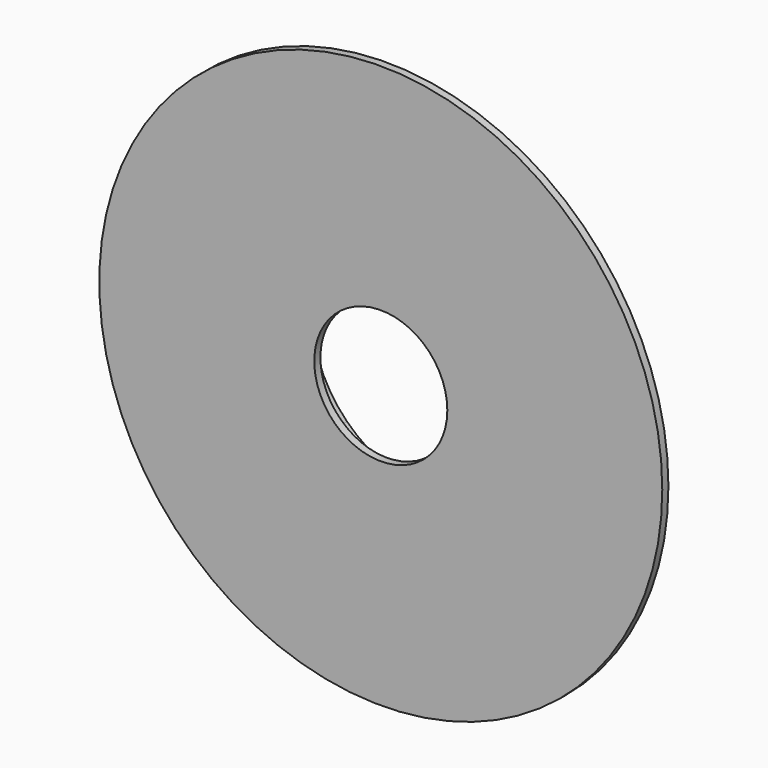
from build123d import *

# Parameters (mm, degrees)
F1_DEPTH = 22
F2_R     = 110
F2_R_2   = 50
F2_R_3   = 47
F3_DEPTH = 3
F4_R     = 26
F5_DEPTH = 3
F6_DEPTH = 25


# Not quite as in the source:
# - a feature names something its author has since deleted; it is built from what else it names


with BuildPart() as f1:
    # F0 (on Front) → F1 (new body)
    with BuildSketch(Plane.XZ):
        with BuildLine():
            Line((48.5, 0), (50, 0))
            ThreePointArc((50, 0), (46.1939766256, 19.1341716183), (35.3553390593, 35.3553390593))
            Line((35.3553390593, 35.3553390593), (34.2946788875, 34.2946788875))
            ThreePointArc((34.2946788875, 34.2946788875), (44.8081573268, 18.5601464697), (48.5, 0))
        make_face()
        with BuildLine():
            ThreePointArc((35.3553390593, -35.3553390593), (46.1939766256, -19.1341716183), (50, 0))
            Line((50, 0), (48.5, 0))
            ThreePointArc((48.5, 0), (44.8081573268, -18.5601464697), (34.2946788875, -34.2946788875))
            Line((34.2946788875, -34.2946788875), (35.3553390593, -35.3553390593))
        make_face()
        with BuildLine():
            Line((34.2946788875, 34.2946788875), (35.3553390593, 35.3553390593))
            ThreePointArc((35.3553390593, 35.3553390593), (19.1341716183, 46.1939766256), (0, 50))
            Line((0, 50), (0, 48.5))
            ThreePointArc((0, 48.5), (18.5601464697, 44.8081573268), (34.2946788875, 34.2946788875))
        make_face()
        with BuildLine():
            ThreePointArc((0, -50), (19.1341716183, -46.1939766256), (35.3553390593, -35.3553390593))
            Line((35.3553390593, -35.3553390593), (34.2946788875, -34.2946788875))
            ThreePointArc((34.2946788875, -34.2946788875), (18.5601464697, -44.8081573268), (0, -48.5))
            Line((0, -48.5), (0, -50))
        make_face()
        with BuildLine():
            Line((47, 0), (48.5, 0))
            ThreePointArc((48.5, 0), (44.8081573268, 18.5601464697), (34.2946788875, 34.2946788875))
            Line((34.2946788875, 34.2946788875), (33.2340187158, 33.2340187158))
            ThreePointArc((33.2340187158, 33.2340187158), (43.422338028, 17.9861213212), (47, 0))
        make_face()
        with BuildLine():
            ThreePointArc((34.2946788875, -34.2946788875), (44.8081573268, -18.5601464697), (48.5, 0))
            Line((48.5, 0), (47, 0))
            ThreePointArc((47, 0), (43.422338028, -17.9861213212), (33.2340187158, -33.2340187158))
            Line((33.2340187158, -33.2340187158), (34.2946788875, -34.2946788875))
        make_face()
        with BuildLine():
            Line((0, 48.5), (0, 50))
            ThreePointArc((0, 50), (-19.1341716183, 46.1939766256), (-35.3553390593, 35.3553390593))
            Line((-35.3553390593, 35.3553390593), (-34.2946788875, 34.2946788875))
            ThreePointArc((-34.2946788875, 34.2946788875), (-18.5601464697, 44.8081573268), (0, 48.5))
        make_face()
        with BuildLine():
            Line((33.2340187158, 33.2340187158), (34.2946788875, 34.2946788875))
            ThreePointArc((34.2946788875, 34.2946788875), (18.5601464697, 44.8081573268), (0, 48.5))
            Line((0, 48.5), (0, 47))
            ThreePointArc((0, 47), (17.9861213212, 43.422338028), (33.2340187158, 33.2340187158))
        make_face()
        with BuildLine():
            ThreePointArc((-35.3553390593, -35.3553390593), (-19.1341716183, -46.1939766256), (0, -50))
            Line((0, -50), (0, -48.5))
            ThreePointArc((0, -48.5), (-18.5601464697, -44.8081573268), (-34.2946788875, -34.2946788875))
            Line((-34.2946788875, -34.2946788875), (-35.3553390593, -35.3553390593))
        make_face()
        with BuildLine():
            ThreePointArc((0, -48.5), (18.5601464697, -44.8081573268), (34.2946788875, -34.2946788875))
            Line((34.2946788875, -34.2946788875), (33.2340187158, -33.2340187158))
            ThreePointArc((33.2340187158, -33.2340187158), (17.9861213212, -43.422338028), (0, -47))
            Line((0, -47), (0, -48.5))
        make_face()
        with BuildLine():
            Line((-34.2946788875, 34.2946788875), (-35.3553390593, 35.3553390593))
            ThreePointArc((-35.3553390593, 35.3553390593), (-46.1939766256, 19.1341716183), (-50, 0))
            Line((-50, 0), (-48.5, 0))
            ThreePointArc((-48.5, 0), (-44.8081573268, 18.5601464697), (-34.2946788875, 34.2946788875))
        make_face()
        with BuildLine():
            Line((0, 47), (0, 48.5))
            ThreePointArc((0, 48.5), (-18.5601464697, 44.8081573268), (-34.2946788875, 34.2946788875))
            Line((-34.2946788875, 34.2946788875), (-33.2340187158, 33.2340187158))
            ThreePointArc((-33.2340187158, 33.2340187158), (-17.9861213212, 43.422338028), (0, 47))
        make_face()
        with BuildLine():
            ThreePointArc((-50, 0), (-46.1939766256, -19.1341716183), (-35.3553390593, -35.3553390593))
            Line((-35.3553390593, -35.3553390593), (-34.2946788875, -34.2946788875))
            ThreePointArc((-34.2946788875, -34.2946788875), (-44.8081573268, -18.5601464697), (-48.5, 0))
            Line((-48.5, 0), (-50, 0))
        make_face()
        with BuildLine():
            ThreePointArc((-34.2946788875, -34.2946788875), (-18.5601464697, -44.8081573268), (0, -48.5))
            Line((0, -48.5), (0, -47))
            ThreePointArc((0, -47), (-17.9861213212, -43.422338028), (-33.2340187158, -33.2340187158))
            Line((-33.2340187158, -33.2340187158), (-34.2946788875, -34.2946788875))
        make_face()
        with BuildLine():
            Line((-33.2340187158, 33.2340187158), (-34.2946788875, 34.2946788875))
            ThreePointArc((-34.2946788875, 34.2946788875), (-44.8081573268, 18.5601464697), (-48.5, 0))
            Line((-48.5, 0), (-47, 0))
            ThreePointArc((-47, 0), (-43.422338028, 17.9861213212), (-33.2340187158, 33.2340187158))
        make_face()
        with BuildLine():
            ThreePointArc((-48.5, 0), (-44.8081573268, -18.5601464697), (-34.2946788875, -34.2946788875))
            Line((-34.2946788875, -34.2946788875), (-33.2340187158, -33.2340187158))
            ThreePointArc((-33.2340187158, -33.2340187158), (-43.422338028, -17.9861213212), (-47, 0))
            Line((-47, 0), (-48.5, 0))
        make_face()
    extrude(amount=F1_DEPTH)

    # F2 (on face) → F3 (join)
    with BuildSketch(Plane.XZ.offset(22)):
        Circle(F2_R)
        Circle(F2_R_2, mode=Mode.SUBTRACT)
        Circle(F2_R_2)
        Circle(F2_R_3, mode=Mode.SUBTRACT)
        Circle(F2_R_3)
    extrude(amount=F3_DEPTH)

    # F4 (on face) → F5 (cut, through all)
    with BuildSketch(Plane.XZ.offset(25)):
        Circle(F4_R)
    extrude(amount=-F5_DEPTH, mode=Mode.SUBTRACT)

    # F0 (on Front) → F6 (join)
    with BuildSketch(Plane.XZ):
        with BuildLine():
            Line((48.5, 0), (50, 0))
            ThreePointArc((50, 0), (46.1939766256, 19.1341716183), (35.3553390593, 35.3553390593))
            Line((35.3553390593, 35.3553390593), (34.2946788875, 34.2946788875))
            ThreePointArc((34.2946788875, 34.2946788875), (44.8081573268, 18.5601464697), (48.5, 0))
        make_face()
        with BuildLine():
            ThreePointArc((35.3553390593, -35.3553390593), (46.1939766256, -19.1341716183), (50, 0))
            Line((50, 0), (48.5, 0))
            ThreePointArc((48.5, 0), (44.8081573268, -18.5601464697), (34.2946788875, -34.2946788875))
            Line((34.2946788875, -34.2946788875), (35.3553390593, -35.3553390593))
        make_face()
        with BuildLine():
            Line((34.2946788875, 34.2946788875), (35.3553390593, 35.3553390593))
            ThreePointArc((35.3553390593, 35.3553390593), (19.1341716183, 46.1939766256), (0, 50))
            Line((0, 50), (0, 48.5))
            ThreePointArc((0, 48.5), (18.5601464697, 44.8081573268), (34.2946788875, 34.2946788875))
        make_face()
        with BuildLine():
            ThreePointArc((0, -50), (19.1341716183, -46.1939766256), (35.3553390593, -35.3553390593))
            Line((35.3553390593, -35.3553390593), (34.2946788875, -34.2946788875))
            ThreePointArc((34.2946788875, -34.2946788875), (18.5601464697, -44.8081573268), (0, -48.5))
            Line((0, -48.5), (0, -50))
        make_face()
        with BuildLine():
            Line((0, 48.5), (0, 50))
            ThreePointArc((0, 50), (-19.1341716183, 46.1939766256), (-35.3553390593, 35.3553390593))
            Line((-35.3553390593, 35.3553390593), (-34.2946788875, 34.2946788875))
            ThreePointArc((-34.2946788875, 34.2946788875), (-18.5601464697, 44.8081573268), (0, 48.5))
        make_face()
        with BuildLine():
            ThreePointArc((-35.3553390593, -35.3553390593), (-19.1341716183, -46.1939766256), (0, -50))
            Line((0, -50), (0, -48.5))
            ThreePointArc((0, -48.5), (-18.5601464697, -44.8081573268), (-34.2946788875, -34.2946788875))
            Line((-34.2946788875, -34.2946788875), (-35.3553390593, -35.3553390593))
        make_face()
        with BuildLine():
            Line((-34.2946788875, 34.2946788875), (-35.3553390593, 35.3553390593))
            ThreePointArc((-35.3553390593, 35.3553390593), (-46.1939766256, 19.1341716183), (-50, 0))
            Line((-50, 0), (-48.5, 0))
            ThreePointArc((-48.5, 0), (-44.8081573268, 18.5601464697), (-34.2946788875, 34.2946788875))
        make_face()
        with BuildLine():
            ThreePointArc((-50, 0), (-46.1939766256, -19.1341716183), (-35.3553390593, -35.3553390593))
            Line((-35.3553390593, -35.3553390593), (-34.2946788875, -34.2946788875))
            ThreePointArc((-34.2946788875, -34.2946788875), (-44.8081573268, -18.5601464697), (-48.5, 0))
            Line((-48.5, 0), (-50, 0))
        make_face()
    extrude(amount=F6_DEPTH)


solid = f1.part
